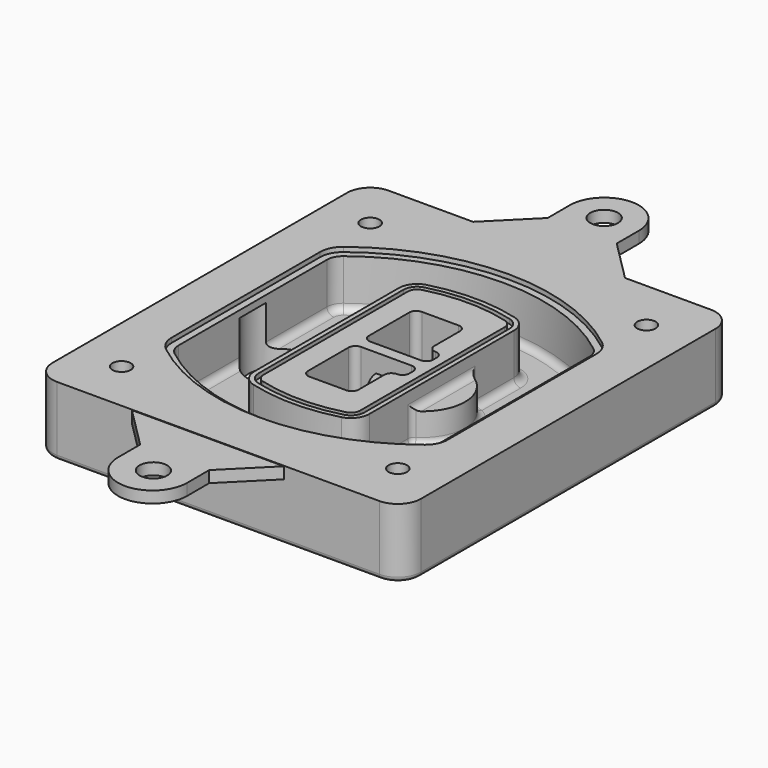
from build123d import *

# Parameters (mm, degrees)
F0_R      = 4
F1_DEPTH  = 25
F2_DEPTH  = 3
F3_DEPTH  = 18
F5_DEPTH  = 21
F6_DEPTH  = 2
F8_DEPTH  = 20
F9_DEPTH  = 16
F10_DEPTH = 25
F7_R      = 6
F7_R_2    = 4
F11_DEPTH = 6
F13_DEPTH = 9
F14_R     = 3
F15_R     = 2
F17_R     = 4
F17_R_2   = 6
F19_DEPTH = 5
F18_R     = 6


# Not quite as in the source:
# - a feature names something its author has since deleted; it is built from what else it names


with BuildPart() as f1:
    # F0 (on Top) → F1 (new body)
    with BuildSketch(Plane.XY):
        with BuildLine():
            ThreePointArc((-80, -80), (-77.0710678119, -87.0710678119), (-70, -90))
            Line((-70, -90), (70, -90))
            ThreePointArc((70, -90), (77.0710678119, -87.0710678119), (80, -80))
            Line((80, -80), (80, 80))
            ThreePointArc((80, 80), (77.0710678119, 87.0710678119), (70, 90))
            Line((70, 90), (-70, 90))
            ThreePointArc((-70, 90), (-77.0710678119, 87.0710678119), (-80, 80))
            Line((-80, 80), (-80, -80))
        make_face()
        with Locations((-60, -67.5)):
            Circle(F0_R, mode=Mode.SUBTRACT)
        with Locations((60, -67.5)):
            Circle(F0_R, mode=Mode.SUBTRACT)
        with Locations((-60, 67.5)):
            Circle(F0_R, mode=Mode.SUBTRACT)
        with BuildLine():
            ThreePointArc((-64, 40.2934422872), (-62.5820384798, 46.4328484224), (-58.6153846154, 51.3286200352))
            ThreePointArc((-58.6153846154, 51.3286200352), (0, 71.5), (58.6153846154, 51.3286200352))
            ThreePointArc((58.6153846154, 51.3286200352), (62.5820384798, 46.4328484224), (64, 40.2934422872))
            Line((64, 40.2934422872), (64, -40.2934422872))
            ThreePointArc((64, -40.2934422872), (62.5820384798, -46.4328484224), (58.6153846154, -51.3286200352))
            ThreePointArc((58.6153846154, -51.3286200352), (0, -71.5), (-58.6153846154, -51.3286200352))
            ThreePointArc((-58.6153846154, -51.3286200352), (-62.5820384798, -46.4328484224), (-64, -40.2934422872))
            Line((-64, -40.2934422872), (-64, 40.2934422872))
        make_face(mode=Mode.SUBTRACT)
        with Locations((60, 67.5)):
            Circle(F0_R, mode=Mode.SUBTRACT)
        with BuildLine():
            ThreePointArc((58.6153846154, 51.3286200352), (0, 71.5), (-58.6153846154, 51.3286200352))
            ThreePointArc((-58.6153846154, 51.3286200352), (-62.5820384798, 46.4328484224), (-64, 40.2934422872))
            Line((-64, 40.2934422872), (-64, -40.2934422872))
            ThreePointArc((-64, -40.2934422872), (-62.5820384798, -46.4328484224), (-58.6153846154, -51.3286200352))
            ThreePointArc((-58.6153846154, -51.3286200352), (0, -71.5), (58.6153846154, -51.3286200352))
            ThreePointArc((58.6153846154, -51.3286200352), (62.5820384798, -46.4328484224), (64, -40.2934422872))
            Line((64, -40.2934422872), (64, 40.2934422872))
            ThreePointArc((64, 40.2934422872), (62.5820384798, 46.4328484224), (58.6153846154, 51.3286200352))
        make_face()
        with BuildLine():
            Line((-60, -40.2934422872), (-60, 40.2934422872))
            ThreePointArc((-60, 40.2934422872), (-58.9871703427, 44.6787323838), (-56.1538461538, 48.1757121072))
            ThreePointArc((-56.1538461538, 48.1757121072), (0, 67.5), (56.1538461538, 48.1757121072))
            ThreePointArc((56.1538461538, 48.1757121072), (58.9871703427, 44.6787323838), (60, 40.2934422872))
            Line((60, 40.2934422872), (60, -40.2934422872))
            ThreePointArc((60, -40.2934422872), (58.9871703427, -44.6787323838), (56.1538461538, -48.1757121072))
            ThreePointArc((56.1538461538, -48.1757121072), (0, -67.5), (-56.1538461538, -48.1757121072))
            ThreePointArc((-56.1538461538, -48.1757121072), (-58.9871703427, -44.6787323838), (-60, -40.2934422872))
        make_face(mode=Mode.SUBTRACT)
        with BuildLine():
            ThreePointArc((-56.1538461538, 48.1757121072), (-58.9871703427, 44.6787323838), (-60, 40.2934422872))
            Line((-60, 40.2934422872), (-60, -40.2934422872))
            ThreePointArc((-60, -40.2934422872), (-58.9871703427, -44.6787323838), (-56.1538461538, -48.1757121072))
            ThreePointArc((-56.1538461538, -48.1757121072), (0, -67.5), (56.1538461538, -48.1757121072))
            ThreePointArc((56.1538461538, -48.1757121072), (58.9871703427, -44.6787323838), (60, -40.2934422872))
            Line((60, -40.2934422872), (60, 40.2934422872))
            ThreePointArc((60, 40.2934422872), (58.9871703427, 44.6787323838), (56.1538461538, 48.1757121072))
            ThreePointArc((56.1538461538, 48.1757121072), (0, 67.5), (-56.1538461538, 48.1757121072))
        make_face()
        with BuildLine():
            ThreePointArc((54.3076923077, 45.8110311612), (56.2910192399, 43.3631453548), (57, 40.2934422872))
            Line((57, 40.2934422872), (57, -40.2934422872))
            ThreePointArc((57, -40.2934422872), (56.2910192399, -43.3631453548), (54.3076923077, -45.8110311612))
            ThreePointArc((54.3076923077, -45.8110311612), (0, -64.5), (-54.3076923077, -45.8110311612))
            ThreePointArc((-54.3076923077, -45.8110311612), (-56.2910192399, -43.3631453548), (-57, -40.2934422872))
            Line((-57, -40.2934422872), (-57, 40.2934422872))
            ThreePointArc((-57, 40.2934422872), (-56.2910192399, 43.3631453548), (-54.3076923077, 45.8110311612))
            ThreePointArc((-54.3076923077, 45.8110311612), (0, 64.5), (54.3076923077, 45.8110311612))
        make_face(mode=Mode.SUBTRACT)
        with BuildLine():
            Line((57, -40.2934422872), (57, 40.2934422872))
            ThreePointArc((57, 40.2934422872), (56.2910192399, 43.3631453548), (54.3076923077, 45.8110311612))
            ThreePointArc((54.3076923077, 45.8110311612), (0, 64.5), (-54.3076923077, 45.8110311612))
            ThreePointArc((-54.3076923077, 45.8110311612), (-56.2910192399, 43.3631453548), (-57, 40.2934422872))
            Line((-57, 40.2934422872), (-57, -40.2934422872))
            ThreePointArc((-57, -40.2934422872), (-56.2910192399, -43.3631453548), (-54.3076923077, -45.8110311612))
            ThreePointArc((-54.3076923077, -45.8110311612), (0, -64.5), (54.3076923077, -45.8110311612))
            ThreePointArc((54.3076923077, -45.8110311612), (56.2910192399, -43.3631453548), (57, -40.2934422872))
        make_face()
    extrude(amount=-F1_DEPTH)

    # F0 (on Top) → F2 (join)
    with BuildSketch(Plane.XY):
        with BuildLine():
            ThreePointArc((-56.1538461538, 48.1757121072), (-58.9871703427, 44.6787323838), (-60, 40.2934422872))
            Line((-60, 40.2934422872), (-60, -40.2934422872))
            ThreePointArc((-60, -40.2934422872), (-58.9871703427, -44.6787323838), (-56.1538461538, -48.1757121072))
            ThreePointArc((-56.1538461538, -48.1757121072), (0, -67.5), (56.1538461538, -48.1757121072))
            ThreePointArc((56.1538461538, -48.1757121072), (58.9871703427, -44.6787323838), (60, -40.2934422872))
            Line((60, -40.2934422872), (60, 40.2934422872))
            ThreePointArc((60, 40.2934422872), (58.9871703427, 44.6787323838), (56.1538461538, 48.1757121072))
            ThreePointArc((56.1538461538, 48.1757121072), (0, 67.5), (-56.1538461538, 48.1757121072))
        make_face()
        with BuildLine():
            ThreePointArc((54.3076923077, 45.8110311612), (56.2910192399, 43.3631453548), (57, 40.2934422872))
            Line((57, 40.2934422872), (57, -40.2934422872))
            ThreePointArc((57, -40.2934422872), (56.2910192399, -43.3631453548), (54.3076923077, -45.8110311612))
            ThreePointArc((54.3076923077, -45.8110311612), (0, -64.5), (-54.3076923077, -45.8110311612))
            ThreePointArc((-54.3076923077, -45.8110311612), (-56.2910192399, -43.3631453548), (-57, -40.2934422872))
            Line((-57, -40.2934422872), (-57, 40.2934422872))
            ThreePointArc((-57, 40.2934422872), (-56.2910192399, 43.3631453548), (-54.3076923077, 45.8110311612))
            ThreePointArc((-54.3076923077, 45.8110311612), (0, 64.5), (54.3076923077, 45.8110311612))
        make_face(mode=Mode.SUBTRACT)
    extrude(amount=F2_DEPTH)

    # F0 (on Top) → F3 (cut)
    with BuildSketch(Plane.XY):
        with BuildLine():
            Line((57, -40.2934422872), (57, 40.2934422872))
            ThreePointArc((57, 40.2934422872), (56.2910192399, 43.3631453548), (54.3076923077, 45.8110311612))
            ThreePointArc((54.3076923077, 45.8110311612), (0, 64.5), (-54.3076923077, 45.8110311612))
            ThreePointArc((-54.3076923077, 45.8110311612), (-56.2910192399, 43.3631453548), (-57, 40.2934422872))
            Line((-57, 40.2934422872), (-57, -40.2934422872))
            ThreePointArc((-57, -40.2934422872), (-56.2910192399, -43.3631453548), (-54.3076923077, -45.8110311612))
            ThreePointArc((-54.3076923077, -45.8110311612), (0, -64.5), (54.3076923077, -45.8110311612))
            ThreePointArc((54.3076923077, -45.8110311612), (56.2910192399, -43.3631453548), (57, -40.2934422872))
        make_face()
    extrude(amount=-F3_DEPTH, mode=Mode.SUBTRACT)

    # F4 (on face) → F5 (join, through all)
    with BuildSketch(Plane.XY.offset(3)):
        with BuildLine():
            ThreePointArc((-25, -39.2465276821), (-23.3511545998, -44.1109737193), (-19.0842911877, -46.9702398883))
            ThreePointArc((-19.0842911877, -46.9702398883), (0, -49.5), (19.0842911877, -46.9702398883))
            ThreePointArc((19.0842911877, -46.9702398883), (23.3511545998, -44.1109737193), (25, -39.2465276821))
            Line((25, -39.2465276821), (25, 39.2465276821))
            ThreePointArc((25, 39.2465276821), (23.3511545998, 44.1109737193), (19.0842911877, 46.9702398883))
            ThreePointArc((19.0842911877, 46.9702398883), (0, 49.5), (-19.0842911877, 46.9702398883))
            ThreePointArc((-19.0842911877, 46.9702398883), (-23.3511545998, 44.1109737193), (-25, 39.2465276821))
            Line((-25, 39.2465276821), (-25, -39.2465276821))
        make_face()
        with BuildLine():
            ThreePointArc((18.5632183908, 45.0393118368), (21.7633659499, 42.89486221), (23, 39.2465276821))
            Line((23, 39.2465276821), (23, -39.2465276821))
            ThreePointArc((23, -39.2465276821), (21.7633659499, -42.89486221), (18.5632183908, -45.0393118368))
            ThreePointArc((18.5632183908, -45.0393118368), (0, -47.5), (-18.5632183908, -45.0393118368))
            ThreePointArc((-18.5632183908, -45.0393118368), (-21.7633659499, -42.89486221), (-23, -39.2465276821))
            Line((-23, -39.2465276821), (-23, 39.2465276821))
            ThreePointArc((-23, 39.2465276821), (-21.7633659499, 42.89486221), (-18.5632183908, 45.0393118368))
            ThreePointArc((-18.5632183908, 45.0393118368), (0, 47.5), (18.5632183908, 45.0393118368))
        make_face(mode=Mode.SUBTRACT)
        with BuildLine():
            Line((23, -39.2465276821), (23, 39.2465276821))
            ThreePointArc((23, 39.2465276821), (21.7633659499, 42.89486221), (18.5632183908, 45.0393118368))
            ThreePointArc((18.5632183908, 45.0393118368), (0, 47.5), (-18.5632183908, 45.0393118368))
            ThreePointArc((-18.5632183908, 45.0393118368), (-21.7633659499, 42.89486221), (-23, 39.2465276821))
            Line((-23, 39.2465276821), (-23, -39.2465276821))
            ThreePointArc((-23, -39.2465276821), (-21.7633659499, -42.89486221), (-18.5632183908, -45.0393118368))
            ThreePointArc((-18.5632183908, -45.0393118368), (0, -47.5), (18.5632183908, -45.0393118368))
            ThreePointArc((18.5632183908, -45.0393118368), (21.7633659499, -42.89486221), (23, -39.2465276821))
        make_face()
        with BuildLine():
            ThreePointArc((18.0421455939, 43.1083837852), (20.1755772999, 41.6787507007), (21, 39.2465276821))
            Line((21, 39.2465276821), (21, -39.2465276821))
            ThreePointArc((21, -39.2465276821), (20.1755772999, -41.6787507007), (18.0421455939, -43.1083837852))
            ThreePointArc((18.0421455939, -43.1083837852), (0, -45.5), (-18.0421455939, -43.1083837852))
            ThreePointArc((-18.0421455939, -43.1083837852), (-20.1755772999, -41.6787507007), (-21, -39.2465276821))
            Line((-21, -39.2465276821), (-21, 39.2465276821))
            ThreePointArc((-21, 39.2465276821), (-20.1755772999, 41.6787507007), (-18.0421455939, 43.1083837852))
            ThreePointArc((-18.0421455939, 43.1083837852), (0, 45.5), (18.0421455939, 43.1083837852))
        make_face(mode=Mode.SUBTRACT)
        with BuildLine():
            Line((21, -39.2465276821), (21, 39.2465276821))
            ThreePointArc((21, 39.2465276821), (20.1755772999, 41.6787507007), (18.0421455939, 43.1083837852))
            ThreePointArc((18.0421455939, 43.1083837852), (0, 45.5), (-18.0421455939, 43.1083837852))
            ThreePointArc((-18.0421455939, 43.1083837852), (-20.1755772999, 41.6787507007), (-21, 39.2465276821))
            Line((-21, 39.2465276821), (-21, -39.2465276821))
            ThreePointArc((-21, -39.2465276821), (-20.1755772999, -41.6787507007), (-18.0421455939, -43.1083837852))
            ThreePointArc((-18.0421455939, -43.1083837852), (0, -45.5), (18.0421455939, -43.1083837852))
            ThreePointArc((18.0421455939, -43.1083837852), (20.1755772999, -41.6787507007), (21, -39.2465276821))
        make_face()
        with BuildLine():
            Line((-8, -2.5), (14, -2.5))
            ThreePointArc((14, -2.5), (16.1213203436, -3.3786796564), (17, -5.5))
            Line((17, -5.5), (17, -7.5))
            ThreePointArc((17, -7.5), (16.1213203436, -9.6213203436), (14, -10.5))
            ThreePointArc((14, -10.5), (11.8786796564, -11.3786796564), (11, -13.5))
            Line((11, -13.5), (11, -27.5))
            ThreePointArc((11, -27.5), (10.1213203436, -29.6213203436), (8, -30.5))
            Line((8, -30.5), (-8, -30.5))
            ThreePointArc((-8, -30.5), (-10.1213203436, -29.6213203436), (-11, -27.5))
            Line((-11, -27.5), (-11, -5.5))
            ThreePointArc((-11, -5.5), (-10.1213203436, -3.3786796564), (-8, -2.5))
        make_face(mode=Mode.SUBTRACT)
        with BuildLine():
            ThreePointArc((-8, 2.5), (-10.1213203436, 3.3786796564), (-11, 5.5))
            Line((-11, 5.5), (-11, 27.5))
            ThreePointArc((-11, 27.5), (-10.1213203436, 29.6213203436), (-8, 30.5))
            Line((-8, 30.5), (8, 30.5))
            ThreePointArc((8, 30.5), (10.1213203436, 29.6213203436), (11, 27.5))
            Line((11, 27.5), (11, 13.5))
            ThreePointArc((11, 13.5), (11.8786796564, 11.3786796564), (14, 10.5))
            ThreePointArc((14, 10.5), (16.1213203436, 9.6213203436), (17, 7.5))
            Line((17, 7.5), (17, 5.5))
            ThreePointArc((17, 5.5), (16.1213203436, 3.3786796564), (14, 2.5))
            Line((14, 2.5), (-8, 2.5))
        make_face(mode=Mode.SUBTRACT)
    extrude(amount=-F5_DEPTH)

    # F4 (on face) → F6 (cut)
    with BuildSketch(Plane.XY.offset(3)):
        with BuildLine():
            Line((23, -39.2465276821), (23, 39.2465276821))
            ThreePointArc((23, 39.2465276821), (21.7633659499, 42.89486221), (18.5632183908, 45.0393118368))
            ThreePointArc((18.5632183908, 45.0393118368), (0, 47.5), (-18.5632183908, 45.0393118368))
            ThreePointArc((-18.5632183908, 45.0393118368), (-21.7633659499, 42.89486221), (-23, 39.2465276821))
            Line((-23, 39.2465276821), (-23, -39.2465276821))
            ThreePointArc((-23, -39.2465276821), (-21.7633659499, -42.89486221), (-18.5632183908, -45.0393118368))
            ThreePointArc((-18.5632183908, -45.0393118368), (0, -47.5), (18.5632183908, -45.0393118368))
            ThreePointArc((18.5632183908, -45.0393118368), (21.7633659499, -42.89486221), (23, -39.2465276821))
        make_face()
        with BuildLine():
            ThreePointArc((18.0421455939, 43.1083837852), (20.1755772999, 41.6787507007), (21, 39.2465276821))
            Line((21, 39.2465276821), (21, -39.2465276821))
            ThreePointArc((21, -39.2465276821), (20.1755772999, -41.6787507007), (18.0421455939, -43.1083837852))
            ThreePointArc((18.0421455939, -43.1083837852), (0, -45.5), (-18.0421455939, -43.1083837852))
            ThreePointArc((-18.0421455939, -43.1083837852), (-20.1755772999, -41.6787507007), (-21, -39.2465276821))
            Line((-21, -39.2465276821), (-21, 39.2465276821))
            ThreePointArc((-21, 39.2465276821), (-20.1755772999, 41.6787507007), (-18.0421455939, 43.1083837852))
            ThreePointArc((-18.0421455939, 43.1083837852), (0, 45.5), (18.0421455939, 43.1083837852))
        make_face(mode=Mode.SUBTRACT)
    extrude(amount=-F6_DEPTH, mode=Mode.SUBTRACT)

    # F7 (on face) → F8 (join)
    with BuildSketch(Plane(origin=(0, 0, -25), x_dir=(1, 0, 0), z_dir=(0, 0, -1))):
        with BuildLine():
            ThreePointArc((3.28842436, 0), (16.7567035675, 13.4682792075), (30.224982775, 0))
            Line((30.224982775, 0), (35.224982775, 0))
            ThreePointArc((35.224982775, 0), (16.7567035675, 18.4682792075), (-1.71157564, 0))
            Line((-1.71157564, 0), (3.28842436, 0))
        make_face()
        with BuildLine():
            Line((3.28842436, 0), (30.224982775, 0))
            ThreePointArc((30.224982775, 0), (16.7567035675, 13.4682792075), (3.28842436, 0))
        make_face()
        with BuildLine():
            ThreePointArc((3.28842436, 0), (16.7567035675, -13.4682792075), (30.224982775, 0))
            Line((30.224982775, 0), (3.28842436, 0))
        make_face()
        with BuildLine():
            Line((35.224982775, 0), (30.224982775, 0))
            ThreePointArc((30.224982775, 0), (16.7567035675, -13.4682792075), (3.28842436, 0))
            Line((3.28842436, 0), (-1.71157564, 0))
            ThreePointArc((-1.71157564, 0), (16.7567035675, -18.4682792075), (35.224982775, 0))
        make_face()
    extrude(amount=-F8_DEPTH)

    # F7 (on face) → F9 (cut)
    with BuildSketch(Plane(origin=(0, 0, -25), x_dir=(1, 0, 0), z_dir=(0, 0, -1))):
        with BuildLine():
            Line((3.28842436, 0), (30.224982775, 0))
            ThreePointArc((30.224982775, 0), (16.7567035675, 13.4682792075), (3.28842436, 0))
        make_face()
        with BuildLine():
            ThreePointArc((3.28842436, 0), (16.7567035675, -13.4682792075), (30.224982775, 0))
            Line((30.224982775, 0), (3.28842436, 0))
        make_face()
    extrude(amount=-F9_DEPTH, mode=Mode.SUBTRACT)

    # F7 (on face) → F10 (cut)
    with BuildSketch(Plane(origin=(0, 0, -25), x_dir=(1, 0, 0), z_dir=(0, 0, -1))):
        with BuildLine():
            Line((-59.0318229325, 0), (-32.0952645175, 0))
            ThreePointArc((-32.0952645175, 0), (-45.563543725, 13.4682792075), (-59.0318229325, 0))
        make_face()
        with BuildLine():
            ThreePointArc((-59.0318229325, 0), (-45.563543725, -13.4682792075), (-32.0952645175, 0))
            Line((-32.0952645175, 0), (-59.0318229325, 0))
        make_face()
    extrude(amount=-F10_DEPTH, mode=Mode.SUBTRACT)

    # F7 (on face) → F11 (cut)
    with BuildSketch(Plane(origin=(0, 0, -25), x_dir=(1, 0, 0), z_dir=(0, 0, -1))):
        with Locations((60, -67.5)):
            Circle(F7_R)
        with Locations((60, -67.5)):
            Circle(F7_R_2, mode=Mode.SUBTRACT)
        with Locations((-60, -67.5)):
            Circle(F7_R)
        with Locations((-60, -67.5)):
            Circle(F7_R_2, mode=Mode.SUBTRACT)
        with Locations((-60, 67.5)):
            Circle(F7_R)
        with Locations((-60, 67.5)):
            Circle(F7_R_2, mode=Mode.SUBTRACT)
        with Locations((60, 67.5)):
            Circle(F7_R)
        with Locations((60, 67.5)):
            Circle(F7_R_2, mode=Mode.SUBTRACT)
    extrude(amount=-F11_DEPTH, mode=Mode.SUBTRACT)

    # F12 (on face) → F13 (cut, through all)
    with BuildSketch(Plane(origin=(0, 0, -9), x_dir=(1, 0, 0), z_dir=(0, 0, -1))):
        with BuildLine():
            Line((11, 13.5), (11, 17.5481537753))
            ThreePointArc((11, 17.5481537753), (2.5696536419, 11.8239143813), (-1.5415842455, 2.5))
            Line((-1.5415842455, 2.5), (3.5224848595, 2.5))
            ThreePointArc((3.5224848595, 2.5), (6.1857188154, 8.3455872281), (11.2536447004, 12.2927168648))
            ThreePointArc((11.2536447004, 12.2927168648), (11.0640958889, 12.8831798879), (11, 13.5))
        make_face()
        with BuildLine():
            ThreePointArc((11.2536447004, -12.2927168648), (6.1857188154, -8.3455872281), (3.5224848595, -2.5))
            Line((3.5224848595, -2.5), (-1.5415842455, -2.5))
            ThreePointArc((-1.5415842455, -2.5), (2.5696536419, -11.8239143813), (11, -17.5481537753))
            Line((11, -17.5481537753), (11, -13.5))
            ThreePointArc((11, -13.5), (11.0640958889, -12.8831798879), (11.2536447004, -12.2927168648))
        make_face()
        with BuildLine():
            ThreePointArc((11.2536447004, 12.2927168648), (6.1857188154, 8.3455872281), (3.5224848595, 2.5))
            Line((3.5224848595, 2.5), (14, 2.5))
            ThreePointArc((14, 2.5), (16.1213203436, 3.3786796564), (17, 5.5))
            Line((17, 5.5), (17, 7.5))
            ThreePointArc((17, 7.5), (16.1213203436, 9.6213203436), (14, 10.5))
            ThreePointArc((14, 10.5), (12.3601599782, 10.9878446101), (11.2536447004, 12.2927168648))
        make_face()
        with BuildLine():
            Line((14, -2.5), (3.5224848595, -2.5))
            ThreePointArc((3.5224848595, -2.5), (6.1857188154, -8.3455872281), (11.2536447004, -12.2927168648))
            ThreePointArc((11.2536447004, -12.2927168648), (12.3601599782, -10.9878446101), (14, -10.5))
            ThreePointArc((14, -10.5), (16.1213203436, -9.6213203436), (17, -7.5))
            Line((17, -7.5), (17, -5.5))
            ThreePointArc((17, -5.5), (16.1213203436, -3.3786796564), (14, -2.5))
        make_face()
    extrude(amount=F13_DEPTH, mode=Mode.SUBTRACT)

    # F14
    f14_edges = [f1.edges().sort_by_distance(p)[0] for p in [
        (-57, -23.703476, -18),
        (-57, 23.703476, -18),
        (25, 0, -5),
        (25, 16.526506, -11.5),
        (25, -16.526506, -11.5),
        (25, -27.886517, -18),
        (35.224983, 0, -18),
    ]]
    fillet(f14_edges, radius=F14_R)

    # F15
    f15_edges = [f1.edges().sort_by_distance(p)[0] for p in [
        (0, -90, -25),
    ]]
    fillet(f15_edges, radius=F15_R)

    # F17 (on face) → F19 (join)
    with BuildSketch(Plane.XY):
        with BuildLine():
            Line((-0.3696787171, 90), (-33.3091765642, 90))
            Line((-33.3091765642, 90), (-70, 90))
            ThreePointArc((-70, 90), (-77.0710678119, 87.0710678119), (-80, 80))
            Line((-80, 80), (-80, -80))
            ThreePointArc((-80, -80), (-77.0710678119, -87.0710678119), (-70, -90))
            Line((-70, -90), (70, -90))
            ThreePointArc((70, -90), (77.0710678119, -87.0710678119), (80, -80))
            Line((80, -80), (80, 80))
            ThreePointArc((80, 80), (77.0710678119, 87.0710678119), (70, 90))
            Line((70, 90), (32.6908234358, 90))
            Line((32.6908234358, 90), (-0.3696787171, 90))
        make_face()
        with Locations((-60, -67.5)):
            Circle(F17_R, mode=Mode.SUBTRACT)
        with Locations((60, -67.5)):
            Circle(F17_R, mode=Mode.SUBTRACT)
        with BuildLine():
            ThreePointArc((-60, 40.2934422872), (-58.9871703427, 44.6787323838), (-56.1538461538, 48.1757121072))
            ThreePointArc((-56.1538461538, 48.1757121072), (0, 67.5), (56.1538461538, 48.1757121072))
            ThreePointArc((56.1538461538, 48.1757121072), (58.9871703427, 44.6787323838), (60, 40.2934422872))
            Line((60, 40.2934422872), (60, -40.2934422872))
            ThreePointArc((60, -40.2934422872), (58.9871703427, -44.6787323838), (56.1538461538, -48.1757121072))
            ThreePointArc((56.1538461538, -48.1757121072), (0, -67.5), (-56.1538461538, -48.1757121072))
            ThreePointArc((-56.1538461538, -48.1757121072), (-58.9871703427, -44.6787323838), (-60, -40.2934422872))
            Line((-60, -40.2934422872), (-60, 40.2934422872))
        make_face(mode=Mode.SUBTRACT)
        with Locations((-60, 67.5)):
            Circle(F17_R, mode=Mode.SUBTRACT)
        with Locations((60, 67.5)):
            Circle(F17_R, mode=Mode.SUBTRACT)
        with BuildLine():
            Line((-15.3091765642, 108), (-33.3091765642, 90))
            Line((-33.3091765642, 90), (-0.3696787171, 90))
            Line((-0.3696787171, 90), (32.6908234358, 90))
            Line((32.6908234358, 90), (14.6908234358, 108))
            Line((14.6908234358, 108), (14.6908234358, 120))
            ThreePointArc((14.6908234358, 120), (-0.3091765642, 135), (-15.3091765642, 120))
            Line((-15.3091765642, 120), (-15.3091765642, 108))
        make_face()
        with Locations((-0.3696787171, 120)):
            Circle(F17_R_2, mode=Mode.SUBTRACT)
    extrude(amount=F19_DEPTH)


with BuildPart() as f19:
    # F18 (on face) → F19, piece 2 (new body)
    with BuildSketch(Plane.XY):
        with BuildLine():
            Line((10.7412714437, -108.3282094902), (28.7412714437, -90.3282094902))
            Line((28.7412714437, -90.3282094902), (-3.897171288, -90.3282094902))
            Line((-3.897171288, -90.3282094902), (-37.2587285563, -90.3282094902))
            Line((-37.2587285563, -90.3282094902), (-19.2587285563, -108.3282094902))
            Line((-19.2587285563, -108.3282094902), (-19.2587285563, -120.3282094902))
            ThreePointArc((-19.2587285563, -120.3282094902), (-4.2587285563, -135.3282094902), (10.7412714437, -120.3282094902))
            Line((10.7412714437, -120.3282094902), (10.7412714437, -108.3282094902))
        make_face()
        with Locations((-3.897171288, -120.3282094902)):
            Circle(F18_R, mode=Mode.SUBTRACT)
    extrude(amount=F19_DEPTH)


solid = Compound([f1.part, f19.part])
